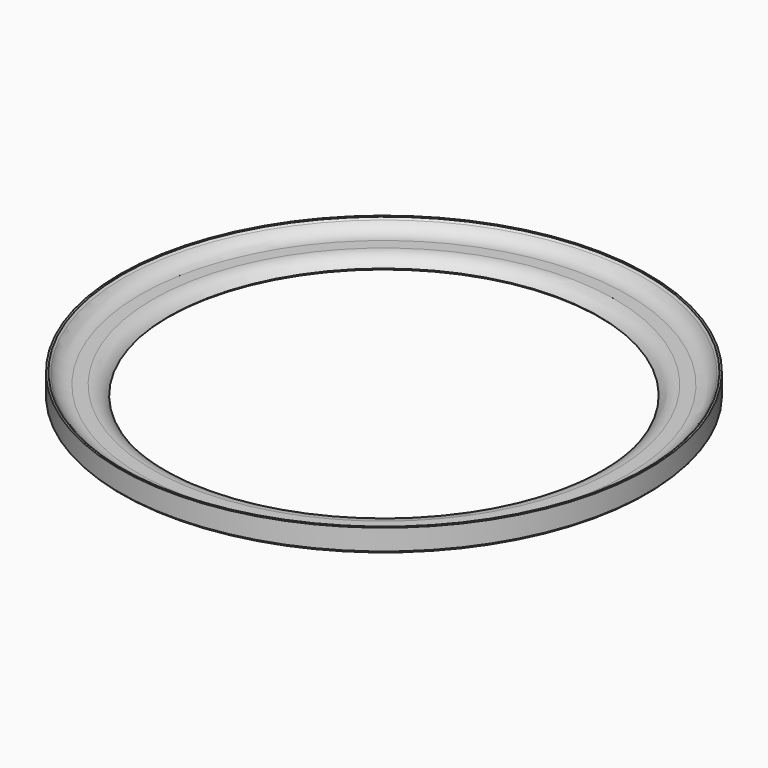
from build123d import *

# Parameters (mm, degrees)
F2_SIZE      = 0.5
F3_TEXT_SIZE = 8.3333333333
F1_FACE1_R   = 69.5
F1_FACE1_R_2 = 69
F4_DEPTH     = 1


# Not quite as in the source:
# - a fillet or chamfer that OpenCascade refuses, or shapes differently, is made with other operations: its cross-section is extruded or revolved along the edge and cut away or added
# - a feature names something its author has since deleted; it is built from what else it names
# - Text() gives the source's letters only with a copy of the font that has no kerning and outlines rounded to 1/6400 em; it was checked with that copy


with BuildPart() as f1:
    # F0 (on Front) → F1 (revolve)
    with BuildSketch(Plane.XZ):
        Polygon((-68.5, 6), (-69.5, 6), (-69.5, 0), (-56.5, 0), (-56.5, 3), (-68.5, 3), align=None)
    revolve(axis=Axis((0, 0, 17.5639875233), (0, 0, -1)))

    # F2
    f2_edges = [f1.edges().sort_by_distance(p)[0] for p in [
        (69.5, 0, 0),
        (56.5, 0, 0),
        (68.5, 0, 6),
    ]]
    chamfer(f2_edges, length=F2_SIZE)

    # F3 (on face) + F1_face1 (on face) → F4 (cut)
    with BuildSketch(Plane(origin=(0, 0, 0), x_dir=(1, 0, 0), z_dir=(0, 0, -1))):
        with Locations((-12.4479166667, 60)):
            Text('98mm', F3_TEXT_SIZE, font='Open Sans', text_align=(TextAlign.LEFT, TextAlign.BOTTOM))
    with BuildSketch(Plane.XY.offset(6)):
        Circle(F1_FACE1_R)
        Circle(F1_FACE1_R_2, mode=Mode.SUBTRACT)
    extrude(amount=-F4_DEPTH, dir=(0, 0, -1), mode=Mode.SUBTRACT)

    # F5: fillet of radius 5 on 2 edges, made by hand

    # F5_s1 → F5_t2 (revolve)
    with BuildSketch(Plane.XZ):
        with BuildLine():
            ThreePointArc((-64.1698729811, 3), (-66.6698729811, 3.6698729811), (-68.5, 5.5))
            Line((-68.5, 5.5), (-68.5, 3))
            Line((-68.5, 3), (-64.1698729811, 3))
        make_face()
    revolve(axis=Axis((0, 0, 3), (0, 0, -1)))

    # F5_s3 → F5_t4 (revolve, cut)
    with BuildSketch(Plane.XZ):
        with BuildLine():
            ThreePointArc((-60.8301270189, 3), (-58.3301270189, 2.3301270189), (-56.5, 0.5))
            Line((-56.5, 0.5), (-56.5, 3))
            Line((-56.5, 3), (-60.8301270189, 3))
        make_face()
    revolve(axis=Axis((0, 0, 3), (0, 0, -1)), mode=Mode.SUBTRACT)


solid = f1.part
